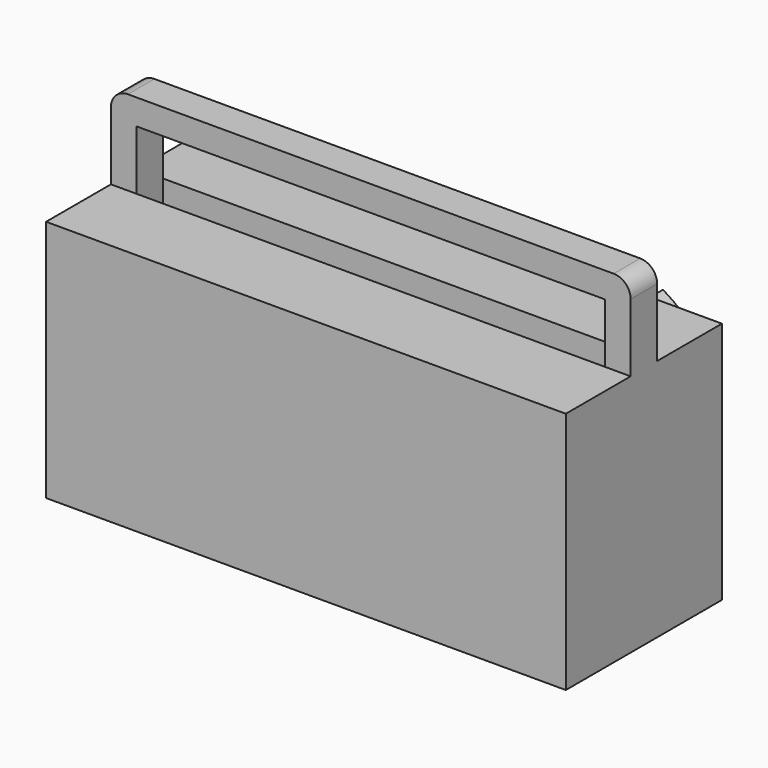
from build123d import *

# Parameters (mm, degrees)
F0_W     = 155.6016728282
F0_H     = 72.8251989931
F1_DEPTH = 58.42
F2_W     = 155.6016728282
F2_H     = 9.92824696
F3_DEPTH = 25.4
F4_T     = 7.62
F5_R     = 5.08
F8_DEPTH = 25.4


# Not quite as in the source:
# - two fillets or chamfers of one size are made in one step
# - a shell that OpenCascade refuses in one call is made with other operations: the cavity is built on its own and cut out


with BuildPart() as f1:
    # F0 (on Front) → F1 (new body)
    with BuildSketch(Plane.XZ):
        with Locations((-1.8093250692, -6.1064558104)):
            Rectangle(F0_W, F0_H)
    extrude(amount=F1_DEPTH)

    # F2 (on face) → F3 (join)
    with BuildSketch(Plane.XY.offset(30.3061436862)):
        with Locations((-1.8093250692, -29.200729914)):
            Rectangle(F2_W, F2_H)
    extrude(amount=F3_DEPTH)

    # F4: shell of thickness 7.62, made by hand


with BuildPart() as f4_core1:
    # F4_t2: copy of F1
    add(f1.part)

    # the walls: a layer under each face that stays
    f4_faces = [f4_core1.faces().sort_by_distance(p)[0] for p in [
        (-1.8093250692, -12.118303217, 30.3061436862),
        (-1.8093250692, 0, -6.1064558104),
        (-79.6101614833, -29.21, 6.5935441896),
        (75.9915113449, -29.21, 6.5935441896),
        (-1.8093250692, -29.21, -42.5190553069),
        (-1.8093250692, -46.292426697, 30.3061436862),
        (-1.8093250692, -58.42, -6.1064558104),
        (-1.8093250692, -29.200729914, 55.7061436862),
    ]]
    thicken(f4_faces, amount=-F4_T, mode=Mode.SUBTRACT)


with BuildPart() as f1_1:
    add(f1.part)

    # what is left inside the walls is the cavity
    f4_cavity = [f4_core1.part.solids().sort_by_distance(p)[0] for p in [
        (-1.809325, -50.7238, -15.703989),
    ]]
    add(f4_cavity, mode=Mode.SUBTRACT)

    # F5
    f5_edges = [f1_1.edges().sort_by_distance(p)[0] for p in [
        (75.991511, -29.20073, 55.706144),
        (-79.610161, -29.20073, 55.706144),
    ]]
    fillet(f5_edges, radius=F5_R)

    # F7 (on face) → F8 (join)
    with BuildSketch(Plane(origin=(0, 0, 0), x_dir=(-1, 0, 0), z_dir=(0, 1, 0))):
        with BuildLine():
            Line((-33.5065312684, 8.8093429804), (-38.0396991968, 16.5818184614))
            ThreePointArc((-38.0396991968, 16.5818184614), (-46.9537485501, -29.5424136332), (0, -31.0426000506))
            ThreePointArc((0, -31.0426000506), (-11.7838373022, -4.7836219306), (-38.2480099797, -16.0991121083))
            ThreePointArc((-38.2480099797, -16.0991121083), (-40.6774615304, -20.5324220373), (-41.8258410886, -25.4556015134))
            ThreePointArc((-41.8258410886, -25.4556015134), (-44.7298971339, -6.6081053321), (-33.5065312684, 8.8093429804))
        make_face()
        with BuildLine():
            ThreePointArc((-31.2344189733, -35.0670516491), (-34.0695631474, -33.473512911), (-36.6739996827, -31.5256118532))
            ThreePointArc((-36.6739996827, -31.5256118532), (-36.1813498713, -25.629843598), (-33.3930179477, -20.4117987305))
            ThreePointArc((-33.3930179477, -20.4117987305), (-24.8135406655, -12.1786870208), (-12.9460245371, -12.9227433354))
            ThreePointArc((-12.9460245371, -12.9227433354), (-6.8355734632, -17.7428655691), (-5.7939905673, -25.4556015134))
            ThreePointArc((-5.7939905673, -25.4556015134), (-16.5679645446, -35.4128057466), (-31.2344189733, -35.0670516491))
        make_face(mode=Mode.SUBTRACT)
    extrude(amount=F8_DEPTH)


solid = f1_1.part
